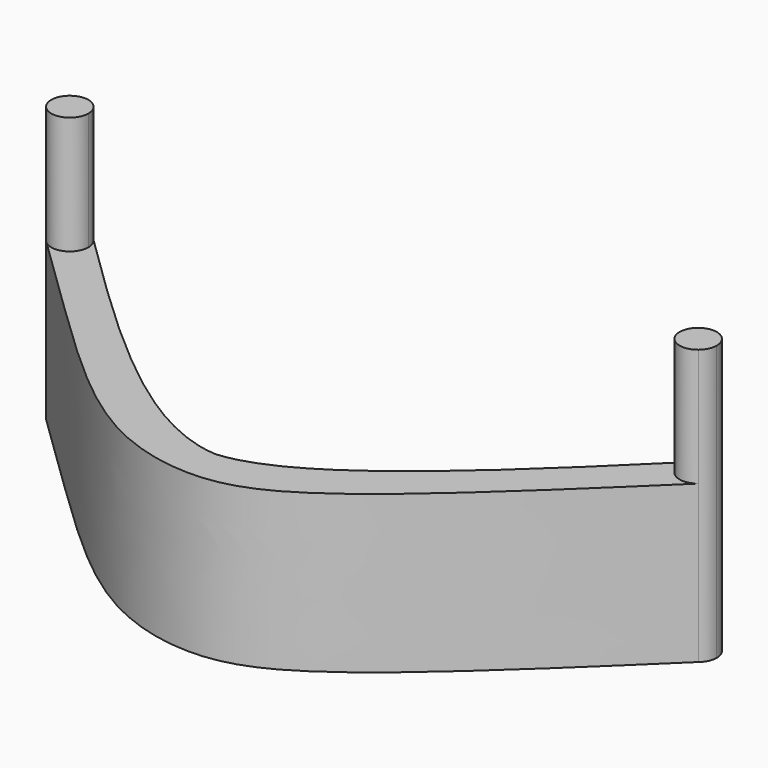
from build123d import *

# Parameters (mm, degrees)
F1_DEPTH = 25.4
F2_DEPTH = 44.45


with BuildPart() as f1:
    # F0 (on Top) → F1 (new body)
    with BuildSketch(Plane.XY):
        with BuildLine():
            add(Edge.make_bspline(
                [(-69.3271539599, -325.7695472874), (-55.2144738249, -339.6916032797), (-40.9515430368, -353.4727855932), (-29.5761530725, -359.1538975577)],
                knots=[0.0032973847, 0.0032973847, 0.0032973847, 0.0032973847, 0.3994432353, 0.3994432353, 0.3994432353, 0.3994432353], degree=3))
            ThreePointArc((-69.3271539599, -325.7695472874), (-68.78999079, -326.6818588732), (-68.6031813399, -327.7239524054))
            ThreePointArc((-68.6031813399, -327.7239524054), (-70.3325433699, -330.4415762111), (-73.526834106, -330.0260297359))
            add(Edge.make_bspline(
                [(-73.526834106, -330.0260297359), (-66.0785739485, -337.1329239072), (-52.6651672252, -350.675327591), (-35.1539032994, -365.4603452904), (-19.3791270617, -369.1866054653), (-3.5859872539, -364.4497262422), (17.9527958908, -343.5527557441), (31.9204714261, -330.0260297359)],
                knots=[0, 0, 0, 0, 0.2194100194, 0.4095312642, 0.5624979229, 0.7156903508, 1, 1, 1, 1], degree=3))
            ThreePointArc((31.9204714261, -330.0260297359), (27.8612970199, -329.8309757381), (27.72079128, -325.7695472874))
            add(Edge.make_bspline(
                [(27.72079128, -325.7695472874), (13.608111145, -339.6916032798), (-0.6548196431, -353.4727855932), (-12.0302096074, -359.1538975577)],
                knots=[0.0032973847, 0.0032973847, 0.0032973847, 0.0032973847, 0.3994432353, 0.3994432353, 0.3994432353, 0.3994432353], degree=3))
            add(Edge.make_bspline(
                [(-20.8031813399, -361.8441262888), (-20.6461461246, -361.8531475586), (-17.281131215, -361.9872858015), (-14.3941104944, -360.8015328656), (-12.0302096074, -359.1538975577)],
                knots=[0.5098577732, 0.5098577732, 0.5098577732, 0.5098577732, 0.5163856275, 0.6506484057, 0.6506484057, 0.6506484057, 0.6506484057], degree=3))
            add(Edge.make_bspline(
                [(-20.8031813399, -361.8441262888), (-20.9602165553, -361.8531475586), (-24.3252314649, -361.9872858015), (-27.2122521855, -360.8015328656), (-29.5761530725, -359.1538975577)],
                knots=[0.5098577732, 0.5098577732, 0.5098577732, 0.5098577732, 0.5163856275, 0.6506484057, 0.6506484057, 0.6506484057, 0.6506484057], degree=3))
        make_face()
        with BuildLine():
            add(Edge.make_bspline(
                [(-29.5761530725, -359.1538975577), (-26.4055823726, -360.7373480762), (-23.4593329293, -361.6915372024), (-20.8031813399, -361.8441262888)],
                knots=[0.3994432353, 0.3994432353, 0.3994432353, 0.3994432353, 0.5098577732, 0.5098577732, 0.5098577732, 0.5098577732], degree=3))
            add(Edge.make_bspline(
                [(-20.8031813399, -361.8441262888), (-20.9602165553, -361.8531475586), (-24.3252314649, -361.9872858015), (-27.2122521855, -360.8015328656), (-29.5761530725, -359.1538975577)],
                knots=[0.5098577732, 0.5098577732, 0.5098577732, 0.5098577732, 0.5163856275, 0.6506484057, 0.6506484057, 0.6506484057, 0.6506484057], degree=3))
        make_face()
        with BuildLine():
            add(Edge.make_bspline(
                [(-12.0302096074, -359.1538975577), (-15.2007803073, -360.7373480762), (-18.1470297506, -361.6915372024), (-20.8031813399, -361.8441262888)],
                knots=[0.3994432353, 0.3994432353, 0.3994432353, 0.3994432353, 0.5098577732, 0.5098577732, 0.5098577732, 0.5098577732], degree=3))
            add(Edge.make_bspline(
                [(-20.8031813399, -361.8441262888), (-20.6461461246, -361.8531475586), (-17.281131215, -361.9872858015), (-14.3941104944, -360.8015328656), (-12.0302096074, -359.1538975577)],
                knots=[0.5098577732, 0.5098577732, 0.5098577732, 0.5098577732, 0.5163856275, 0.6506484057, 0.6506484057, 0.6506484057, 0.6506484057], degree=3))
        make_face()
    extrude(amount=F1_DEPTH)

    # F0 (on Top) → F2 (join)
    with BuildSketch(Plane.XY):
        with BuildLine():
            Line((28.073165894, -325.4218750749), (31.9204714261, -330.0260297359))
            ThreePointArc((31.9204714261, -330.0260297359), (32.7144424657, -328.9945903755), (32.9968186601, -327.7239524054))
            ThreePointArc((32.9968186601, -327.7239524054), (31.2674566301, -325.0063285998), (28.073165894, -325.4218750749))
        make_face()
        with BuildLine():
            ThreePointArc((27.72079128, -325.7695472874), (27.8612970199, -329.8309757381), (31.9204714261, -330.0260297359))
            Line((31.9204714261, -330.0260297359), (28.073165894, -325.4218750749))
            add(Edge.make_bspline(
                [(28.073165894, -325.4218750749), (27.9557192671, -325.5377725126), (27.8382604785, -325.6536647801), (27.72079128, -325.7695472874)],
                knots=[0, 0, 0, 0, 0.0032973847, 0.0032973847, 0.0032973847, 0.0032973847], degree=3))
        make_face()
        with BuildLine():
            add(Edge.make_bspline(
                [(-69.6795285739, -325.4218750749), (-69.562081947, -325.5377725126), (-69.4446231584, -325.6536647801), (-69.3271539599, -325.7695472874)],
                knots=[0, 0, 0, 0, 0.0032973847, 0.0032973847, 0.0032973847, 0.0032973847], degree=3))
            Line((-69.6795285739, -325.4218750749), (-73.526834106, -330.0260297359))
            ThreePointArc((-73.526834106, -330.0260297359), (-70.3325433699, -330.4415762111), (-68.6031813399, -327.7239524054))
            ThreePointArc((-68.6031813399, -327.7239524054), (-68.78999079, -326.6818588732), (-69.3271539599, -325.7695472874))
        make_face()
        with BuildLine():
            Line((-73.526834106, -330.0260297359), (-69.6795285739, -325.4218750749))
            ThreePointArc((-69.6795285739, -325.4218750749), (-73.9052586704, -325.8002996394), (-73.526834106, -330.0260297359))
        make_face()
    extrude(amount=F2_DEPTH)


solid = f1.part
